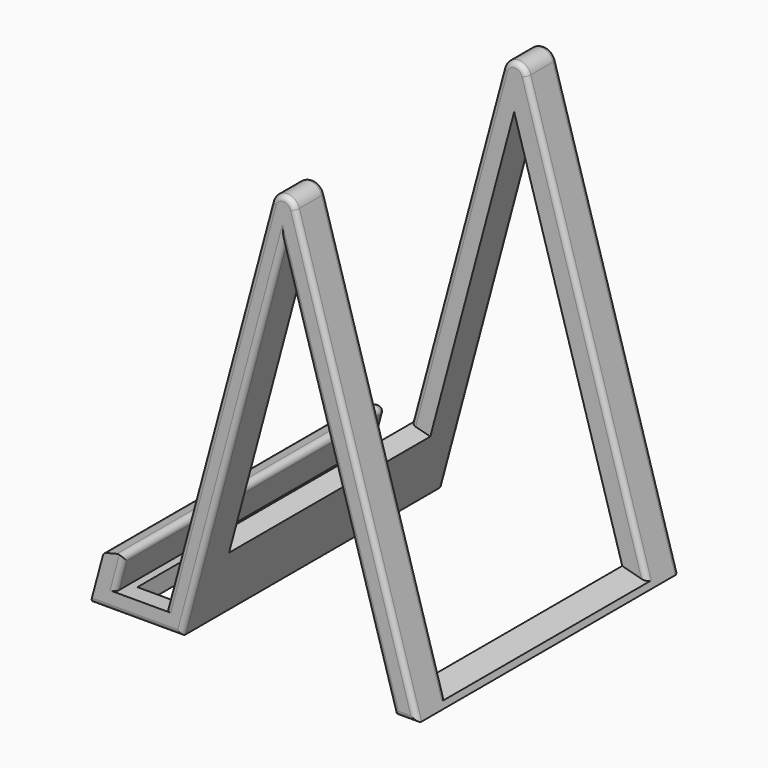
from build123d import *

# Parameters (mm, degrees)
F1_DEPTH    = 130
F2_R        = 2
F3_T1_DEPTH = 130
F3_T4_ANGLE = 148.4890190499
F3_T6_ANGLE = 148.4890190499
F4_W        = 18
F4_H        = 116
F5_DEPTH    = 15
F6_W        = 100
F6_H        = 140.9174852884
F6_H_2      = 11.4719050156
F1_FACE2_W  = 126
F1_FACE2_H  = 170.8886996293
F7_DEPTH    = 300
F8_R        = 2


# Not quite as in the source:
# - a fillet or chamfer that OpenCascade refuses, or shapes differently, is made with other operations: its cross-section is extruded or revolved along the edge and cut away or added


with BuildPart() as f1:
    # F0 (on Front) → F1 (new body)
    with BuildSketch(Plane.XZ):
        Polygon((-46.5874281185, -17.2704798563), (-66.5874281185, -17.2704798563), (-62.7051424419, -2.781592462), (-71.2205818073, -4.9188610433), (-76.3969627094, -24.2373775691), (-40.1931625425, -24.2373775691), (0, 125.7655471563), (44.4641634577, -24.2373775691), (53.6030372906, -24.2373775691), (0, 156.5961688757), align=None)
    extrude(amount=F1_DEPTH)

    # F2
    f2_edges = [f1.edges().sort_by_distance(p)[0] for p in [
        (-23.293714, -130, 69.662845),
        (-20.096581, -130, 50.764085),
        (-64.646285, -130, -10.026036),
        (-62.705142, -65, -2.781592),
        (-71.220582, -65, -4.918861),
        (22.232082, -130, 50.764085),
        (26.801519, -130, 66.179396),
        (-23.293714, 0, 69.662845),
        (-20.096581, 0, 50.764085),
        (-56.587428, 0, -17.27048),
        (-64.646285, 0, -10.026036),
        (-66.962862, 0, -3.850227),
        (-73.808772, 0, -14.578119),
        (-58.295063, 0, -24.237378),
        (22.232082, 0, 50.764085),
        (49.0336, 0, -24.237378),
        (26.801519, 0, 66.179396),
        (-58.295063, -130, -24.237378),
        (49.0336, -130, -24.237378),
    ]]
    fillet(f2_edges, radius=F2_R)

    # F3: fillet of radius 5 on 1 edges, made by hand

    # F3_s2 → F3_t1 (cut)
    with BuildSketch(Plane.XZ):
        with BuildLine():
            ThreePointArc((-4.5868330474, 139.4778748971), (0.1768690132, 143.1833450148), (5.0366225074, 139.6047751759))
            Line((5.0366225074, 139.6047751759), (0, 156.5961688757))
            Line((0, 156.5961688757), (-4.5868330474, 139.4778748971))
        make_face()
    extrude(amount=F3_T1_DEPTH, mode=Mode.SUBTRACT)

    # F3_s3 → F3_t4 (revolve, cut)
    with BuildSketch(Plane(origin=(34.5622091716, 0, 128.9879206501), x_dir=(0, 1, 0), z_dir=(-0.2588190451, 0, -0.9659258263))):
        with BuildLine():
            ThreePointArc((0, -38.5300708951), (-0.5857864376, -39.9442844575), (-2, -40.5300708951))
            Line((-2, -40.5300708951), (0, -40.5300708951))
            Line((0, -40.5300708951), (0, -38.5300708951))
        make_face()
    revolve(axis=Axis((0.2427960841, 0, 138.1837796716), (0, 1, 0)), revolution_arc=F3_T4_ANGLE, mode=Mode.SUBTRACT)

    # F3_s5 → F3_t6 (revolve, cut)
    with BuildSketch(Plane(origin=(-37.6327378938, 0, 126.9566390213), x_dir=(0, 1, 0), z_dir=(0.2841991009, 0, -0.9587652847))):
        with BuildLine():
            ThreePointArc((-130, 42.5044903939), (-129.4142135624, 43.9187039563), (-128, 44.5044903939))
            Line((-128, 44.5044903939), (-130, 44.5044903939))
            Line((-130, 44.5044903939), (-130, 42.5044903939))
        make_face()
    revolve(axis=Axis((0.2427960841, -130, 138.1837796716), (0, -1, 0)), revolution_arc=F3_T6_ANGLE, mode=Mode.SUBTRACT)

    # F4 (on face) → F5 (cut)
    with BuildSketch(Plane(origin=(0, 0, -24.2373775691), x_dir=(1, 0, 0), z_dir=(0, 0, -1))):
        with Locations((-54.3969627094, 65)):
            Rectangle(F4_W, F4_H)
    extrude(amount=-F5_DEPTH, mode=Mode.SUBTRACT)

    # F6 (on face) + F1_face2 (on face) → F7 (cut)
    with BuildSketch(Plane(origin=(-39.1490422189, 0, 10.489954247), x_dir=(0, -1, 0), z_dir=(-0.9659258263, 0, 0.2588190451))):
        with Locations((65, 63.0793791654)):
            Rectangle(F6_W, F6_H)
        with Locations((65, 139.2740743175)):
            Rectangle(F6_W, F6_H_2)
    with BuildSketch(Plane(origin=(29.319829899, -65, 57.6836988034), x_dir=(0, 1, 0), z_dir=(0.9587652847, 0, 0.2841991009))):
        Rectangle(F1_FACE2_W, F1_FACE2_H)
    extrude(amount=-F7_DEPTH, dir=(-0.9659258263, 0, 0.2588190451), mode=Mode.SUBTRACT)

    # F8
    f8_edges = [f1.edges().sort_by_distance(p)[0] for p in [
        (-22.822898, -15, 71.419956),
        (28.960029, -115, 58.897511),
        (-22.822898, -115, 71.419956),
        (0.176869, -115, 143.183345),
        (28.960029, -15, 58.897511),
        (0.176869, -15, 143.183345),
    ]]
    fillet(f8_edges, radius=F8_R)


solid = f1.part
